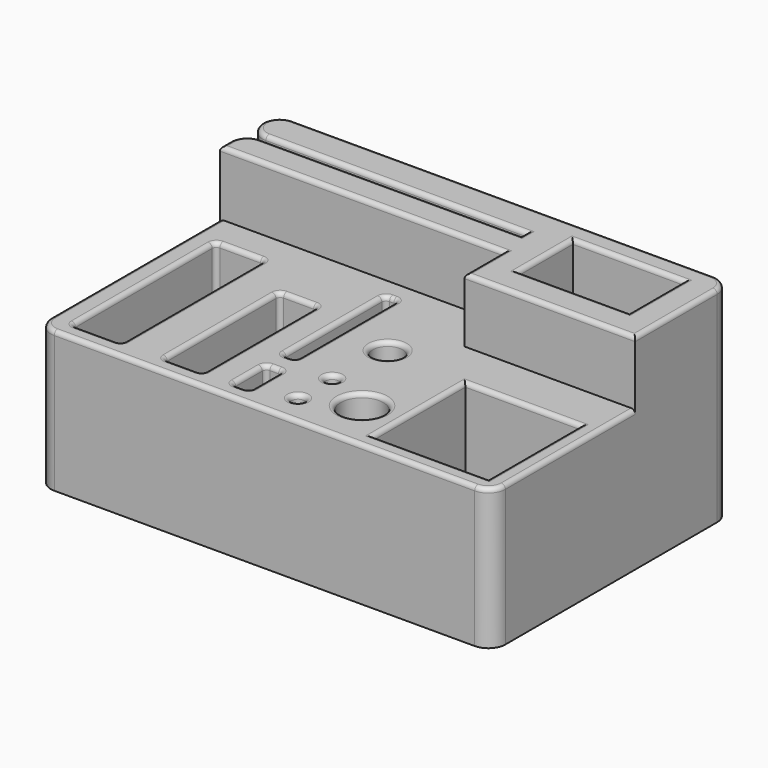
from build123d import *

# Parameters (mm, degrees)
F0_W         = 106.5
F0_H         = 70
F1_DEPTH     = 3
F2_W         = 4
F2_H         = 9.8
F2_W_2       = 11.5
F2_H_2       = 42
F2_W_3       = 9
F2_H_3       = 33.8
F2_W_4       = 3
F2_H_4       = 30
F2_R         = 1.5
F2_R_2       = 5
F2_R_3       = 3.5
F2_W_5       = 27
F2_H_5       = 27
F3_DEPTH     = 30
F2_W_6       = 26
F2_H_6       = 16
F4_DEPTH     = 45
F5_R         = 1
F6_T1_DEPTH  = 43
F6_T3_DEPTH  = 58
F6_T5_DEPTH  = 45
F6_T8_ANGLE  = 90
F6_T10_ANGLE = 90
F6_T12_ANGLE = 90
F6_T14_ANGLE = 90
F6_T16_ANGLE = 90
F6_T18_ANGLE = 90


# Not quite as in the source:
# - a fillet or chamfer that OpenCascade refuses, or shapes differently, is made with other operations: its cross-section is extruded or revolved along the edge and cut away or added


with BuildPart() as f1:
    # F0 (on Top) → F1 (new body)
    with BuildSketch(Plane.XY):
        Rectangle(F0_W, F0_H)
    extrude(amount=F1_DEPTH)

    # F2 (on face) → F3 (join)
    with BuildSketch(Plane.XY.offset(3)):
        Polygon((13.25, 18.5), (-53.25, 18.5), (-53.25, -35), (53.25, -35), (53.25, 7), (13.25, 7), align=None)
        with Locations((-8.75, -26.1)):
            Rectangle(F2_W, F2_H, mode=Mode.SUBTRACT)
        with Locations((-42.5, -10)):
            Rectangle(F2_W_2, F2_H_2, mode=Mode.SUBTRACT)
        with Locations((-22.25, -14.1)):
            Rectangle(F2_W_3, F2_H_3, mode=Mode.SUBTRACT)
        with Locations((-9.25, -1.2)):
            Rectangle(F2_W_4, F2_H_4, mode=Mode.SUBTRACT)
        with Locations((2.25, -28)):
            Circle(F2_R, mode=Mode.SUBTRACT)
        with Locations((13.25, -23)):
            Circle(F2_R_2, mode=Mode.SUBTRACT)
        with Locations((2.25, -18)):
            Circle(F2_R, mode=Mode.SUBTRACT)
        with Locations((3.25, -3)):
            Circle(F2_R_3, mode=Mode.SUBTRACT)
        with Locations((35.75, -17.5)):
            Rectangle(F2_W_5, F2_H_5, mode=Mode.SUBTRACT)
    extrude(amount=F3_DEPTH)

    # F2 (on face) → F4 (join)
    with BuildSketch(Plane.XY.offset(3)):
        Polygon((-53.25, 35), (-53.25, 27), (11.75, 27), (11.75, 25.5), (-53.25, 25.5), (-53.25, 18.5), (13.25, 18.5), (13.25, 7), (53.25, 7), (53.25, 35), align=None)
        with Locations((33.25, 22)):
            Rectangle(F2_W_6, F2_H_6, mode=Mode.SUBTRACT)
    extrude(amount=F4_DEPTH)

    # F5
    f5_edges = [f1.edges().sort_by_distance(p)[0] for p in [
        (8.25, -23, 33),
        (35.75, -4, 33),
        (22.25, -17.5, 33),
        (49.25, -17.5, 33),
        (35.75, -31, 33),
        (0.75, -18, 33),
        (-0.25, -3, 33),
        (0.75, -28, 33),
        (-0.25, -3, 3),
        (0.75, -28, 3),
        (0.75, -18, 3),
        (-7.75, -1.2, 33),
        (-6.75, -26.1, 33),
        (-10.75, -1.2, 33),
        (-10.75, -26.1, 33),
        (-9.25, 13.8, 33),
        (-6.75, -21.2, 18),
        (-7.75, -16.2, 18),
        (-8.75, -31, 33),
        (-10.75, -21.2, 18),
        (-9.25, -16.2, 33),
        (-8.75, -21.2, 33),
        (-7.75, -1.2, 3),
        (-8.75, -31, 3),
        (-10.75, -31, 18),
        (-8.75, -21.2, 3),
        (-6.75, -31, 18),
        (-10.75, -26.1, 3),
        (-9.25, 13.8, 3),
        (-10.75, -16.2, 18),
        (-7.75, 13.8, 18),
        (-10.75, -1.2, 3),
        (-10.75, 13.8, 18),
        (-6.75, -26.1, 3),
        (-9.25, -16.2, 3),
        (-17.75, -14.1, 33),
        (-26.75, -14.1, 33),
        (-22.25, -31, 33),
        (-22.25, 2.8, 33),
        (-17.75, -14.1, 3),
        (-26.75, -14.1, 3),
        (-26.75, 2.8, 18),
        (-17.75, -31, 18),
        (-26.75, -31, 18),
        (-22.25, -31, 3),
        (-22.25, 2.8, 3),
        (-17.75, 2.8, 18),
        (-36.75, -10, 33),
        (-48.25, -10, 33),
        (-42.5, -31, 33),
        (-42.5, 11, 33),
        (-36.75, -10, 3),
        (-48.25, -10, 3),
        (-48.25, 11, 18),
        (-36.75, -31, 18),
        (-36.75, 11, 18),
        (-48.25, -31, 18),
        (-42.5, 11, 3),
        (-42.5, -31, 3),
        (-53.25, -8.25, 33),
        (0, -35, 33),
        (53.25, -14, 33),
        (-20, 18.5, 48),
        (13.25, 12.75, 48),
        (33.25, 7, 48),
        (53.25, 21, 48),
        (0, 35, 48),
        (-53.25, 31, 48),
        (-53.25, 22, 48),
        (-20.75, 27, 48),
        (11.75, 26.25, 48),
        (-20.75, 25.5, 48),
        (20.25, 22, 48),
        (33.25, 30, 48),
        (46.25, 22, 48),
        (33.25, 14, 48),
    ]]
    fillet(f5_edges, radius=F5_R)

    # F6: fillet of radius 4 on 6 edges, made by hand

    # F6_s2 → F6_t1 (cut)
    with BuildSketch(Plane.XY.offset(-10)):
        with BuildLine():
            ThreePointArc((53.25, -31), (52.0784271247, -33.8284271247), (49.25, -35))
            Line((49.25, -35), (53.25, -35))
            Line((53.25, -35), (53.25, -31))
        make_face()
        with BuildLine():
            ThreePointArc((-53.25, -31), (-52.0784271247, -33.8284271247), (-49.25, -35))
            Line((-49.25, -35), (-53.25, -35))
            Line((-53.25, -35), (-53.25, -31))
        make_face()
    extrude(amount=F6_T1_DEPTH, mode=Mode.SUBTRACT)

    # F6_s4 → F6_t3 (cut)
    with BuildSketch(Plane.XY.offset(-10)):
        with BuildLine():
            ThreePointArc((-49.25, 35), (-52.0784271247, 33.8284271247), (-53.25, 31))
            Line((-53.25, 31), (-53.25, 35))
            Line((-53.25, 35), (-49.25, 35))
        make_face()
        with BuildLine():
            ThreePointArc((49.25, 35), (52.0784271247, 33.8284271247), (53.25, 31))
            Line((53.25, 31), (53.25, 35))
            Line((53.25, 35), (49.25, 35))
        make_face()
    extrude(amount=F6_T3_DEPTH, mode=Mode.SUBTRACT)

    # F6_s6 → F6_t5 (cut)
    with BuildSketch(Plane.XY.offset(3)):
        with BuildLine():
            ThreePointArc((-53.25, 21.5), (-52.0784271247, 24.3284271247), (-49.25, 25.5))
            Line((-49.25, 25.5), (-53.25, 25.5))
            Line((-53.25, 25.5), (-53.25, 21.5))
        make_face()
        with BuildLine():
            ThreePointArc((-53.25, 31), (-52.0784271247, 28.1715728753), (-49.25, 27))
            Line((-49.25, 27), (-53.25, 27))
            Line((-53.25, 27), (-53.25, 31))
        make_face()
    extrude(amount=F6_T5_DEPTH, mode=Mode.SUBTRACT)

    # F6_s7 → F6_t8 (revolve, cut)
    with BuildSketch(Plane.XZ.offset(-31)):
        with BuildLine():
            ThreePointArc((-52.25, 48), (-52.9571067812, 47.7071067812), (-53.25, 47))
            Line((-53.25, 47), (-53.25, 48))
            Line((-53.25, 48), (-52.25, 48))
        make_face()
    revolve(axis=Axis((-49.25, 31, 48), (0, 0, 1)), revolution_arc=F6_T8_ANGLE, mode=Mode.SUBTRACT)

    # F6_s9 → F6_t10 (revolve, cut)
    with BuildSketch(Plane.YZ.offset(-49.25)):
        with BuildLine():
            ThreePointArc((24.5, 48), (25.2071067812, 47.7071067812), (25.5, 47))
            Line((25.5, 47), (25.5, 48))
            Line((25.5, 48), (24.5, 48))
        make_face()
    revolve(axis=Axis((-49.25, 21.5, 48), (0, 0, 1)), revolution_arc=F6_T10_ANGLE, mode=Mode.SUBTRACT)

    # F6_s11 → F6_t12 (revolve, cut)
    with BuildSketch(Plane.XZ.offset(-31)):
        with BuildLine():
            ThreePointArc((52.25, 48), (52.9571067812, 47.7071067812), (53.25, 47))
            Line((53.25, 47), (53.25, 48))
            Line((53.25, 48), (52.25, 48))
        make_face()
    revolve(axis=Axis((49.25, 31, 48), (0, 0, 1)), revolution_arc=F6_T12_ANGLE, mode=Mode.SUBTRACT)

    # F6_s13 → F6_t14 (revolve, cut)
    with BuildSketch(Plane.YZ.offset(-49.25)):
        with BuildLine():
            ThreePointArc((34, 48), (34.7071067812, 47.7071067812), (35, 47))
            Line((35, 47), (35, 48))
            Line((35, 48), (34, 48))
        make_face()
    revolve(axis=Axis((-49.25, 31, 48), (0, 0, 1)), revolution_arc=F6_T14_ANGLE, mode=Mode.SUBTRACT)

    # F6_s15 → F6_t16 (revolve, cut)
    with BuildSketch(Plane.XZ.offset(31)):
        with BuildLine():
            ThreePointArc((-52.25, 33), (-52.9571067812, 32.7071067812), (-53.25, 32))
            Line((-53.25, 32), (-53.25, 33))
            Line((-53.25, 33), (-52.25, 33))
        make_face()
    revolve(axis=Axis((-49.25, -31, 33), (0, 0, 1)), revolution_arc=F6_T16_ANGLE, mode=Mode.SUBTRACT)

    # F6_s17 → F6_t18 (revolve, cut)
    with BuildSketch(Plane.YZ.offset(49.25)):
        with BuildLine():
            ThreePointArc((-34, 33), (-34.7071067812, 32.7071067812), (-35, 32))
            Line((-35, 32), (-35, 33))
            Line((-35, 33), (-34, 33))
        make_face()
    revolve(axis=Axis((49.25, -31, 33), (0, 0, 1)), revolution_arc=F6_T18_ANGLE, mode=Mode.SUBTRACT)


solid = f1.part
